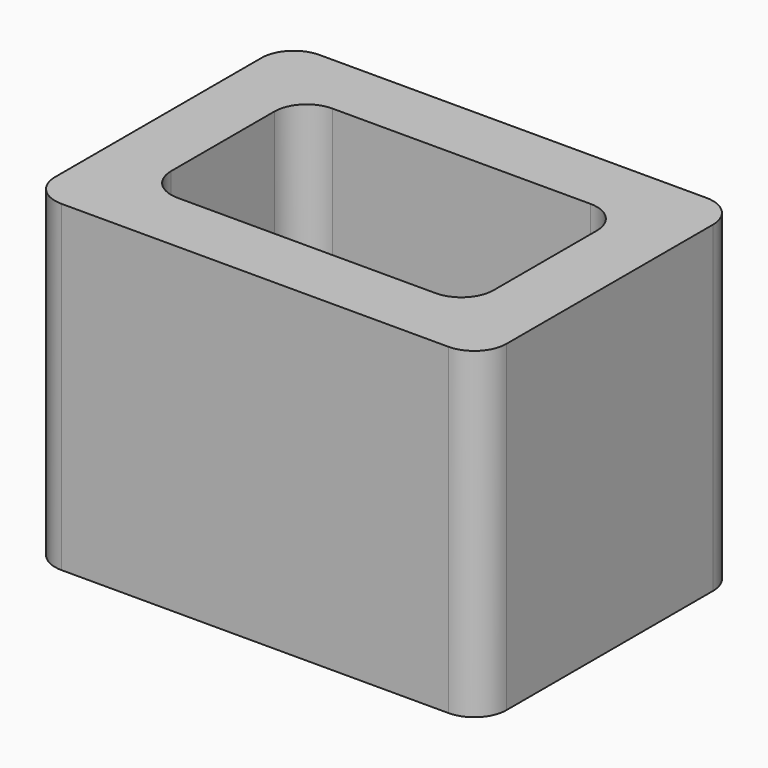
from build123d import *

# Parameters (mm, degrees)
F0_W     = 177.8
F0_H     = 127
F1_DEPTH = 127
F2_T     = -25.4
F3_R     = 12.7


with BuildPart() as f1:
    # F0 (on Top) → F1 (new body)
    with BuildSketch(Plane.XY):
        with Locations((88.9, -63.5)):
            Rectangle(F0_W, F0_H)
    extrude(amount=F1_DEPTH)

    # F2
    f2_openings = [f1.faces().sort_by_distance(p)[0] for p in [
        (88.9, -63.5, 127),
    ]]
    offset(amount=F2_T, openings=f2_openings)

    # F3
    f3_edges = [f1.edges().sort_by_distance(p)[0] for p in [
        (152.4, -101.6, 76.2),
        (88.9, -101.6, 25.4),
        (25.4, -101.6, 76.2),
        (25.4, -25.4, 76.2),
        (25.4, -63.5, 25.4),
        (88.9, -25.4, 25.4),
        (152.4, -25.4, 76.2),
        (152.4, -63.5, 25.4),
        (177.8, 0, 63.5),
        (177.8, -127, 63.5),
        (0, -127, 63.5),
        (0, 0, 63.5),
    ]]
    fillet(f3_edges, radius=F3_R)


solid = f1.part
